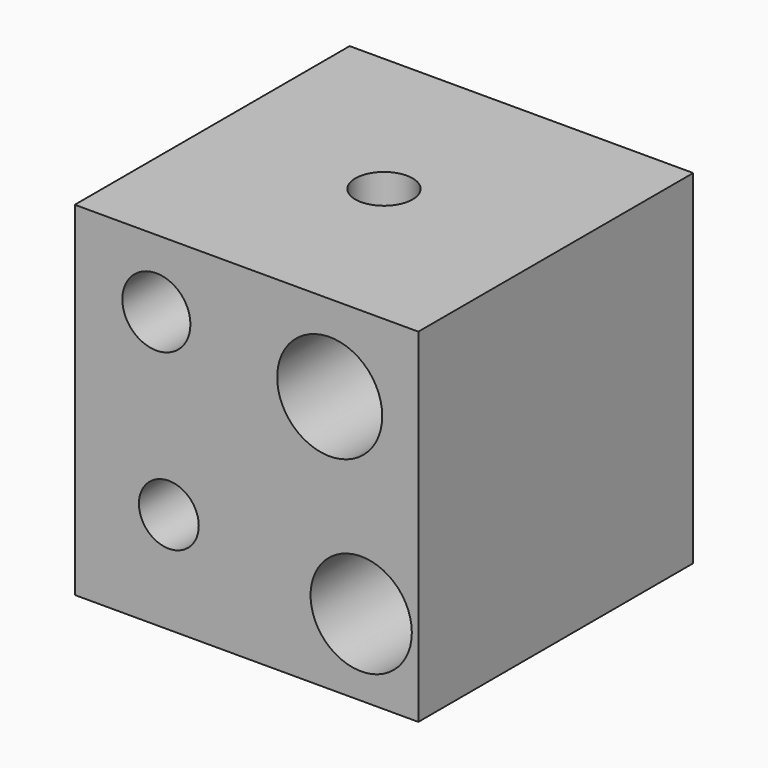
from build123d import *

# Parameters (mm, degrees)
F0_W     = 152.4
F0_H     = 152.4
F0_R     = 12.7
F1_DEPTH = 152.4
F2_R     = 15.0984188398
F2_R_2   = 23.2988824092
F2_R_3   = 22.4609439984
F2_R_4   = 13.2743249865
F3_DEPTH = 152.401


# Not quite as in the source:
# - the program builds the solid bodies; features that only make, move or delete a surface that nothing else refers to are left out


with BuildPart() as f1:
    # F0 (on Top) → F1 (new body)
    with BuildSketch(Plane.XY):
        Rectangle(F0_W, F0_H)
        Circle(F0_R, mode=Mode.SUBTRACT)
    extrude(amount=F1_DEPTH)

    # F2 (on face) → F3 (cut, through all)
    with BuildSketch(Plane.XZ.offset(76.2)):
        with Locations((-40.0141887367, 122.3329827189)):
            Circle(F2_R)
        with Locations((36.8730016053, 114.2153069377)):
            Circle(F2_R_2)
        with Locations((50.8471243083, 33.929079771)):
            Circle(F2_R_3)
        with Locations((-34.4802364707, 44.915728271)):
            Circle(F2_R_4)
    extrude(amount=-F3_DEPTH, mode=Mode.SUBTRACT)


solid = f1.part
